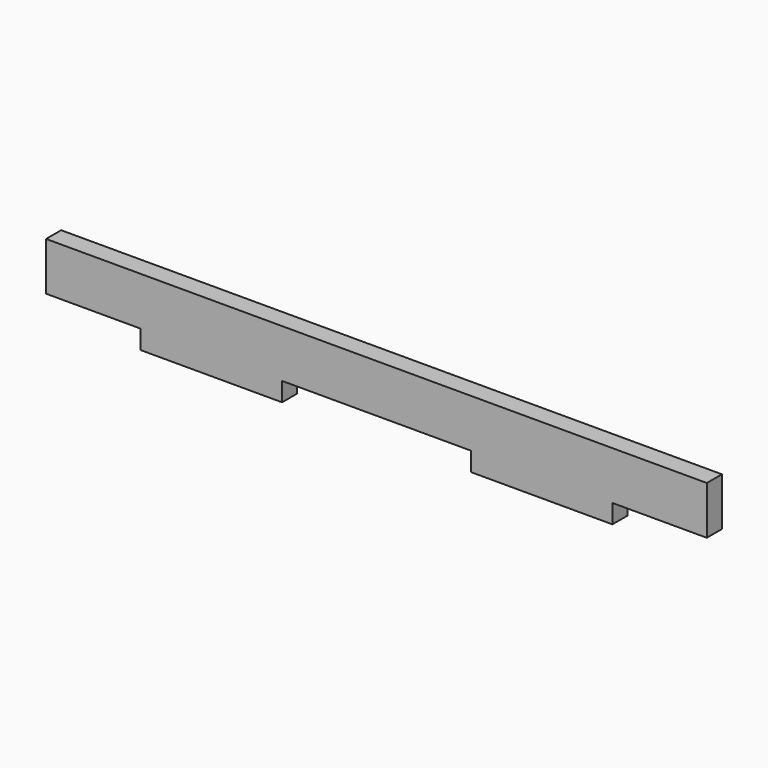
from build123d import *

# Parameters (mm, degrees)
F1_DEPTH = 5.08


# Not quite as in the source:
# - a feature names something its author has since deleted; it is built from what else it names


with BuildPart() as f1:
    # F0 (on Front) → F1 (new body)
    with BuildSketch(Plane.XZ):
        Polygon((-25.4, 0), (0, 0), (25.4, 0), (25.4, -5.08), (63.5, -5.08), (63.5, 0), (88.9, 0), (88.9, 3.1722693238), (88.9, 6.3445386477), (88.9, 12.9838371649), (-88.9, 12.9838371649), (-88.9, 6.3445386477), (-88.9, 3.1722693238), (-88.9, 0), (-63.5, 0), (-63.5, -5.08), (-25.4, -5.08), align=None)
    extrude(amount=F1_DEPTH)


solid = f1.part
